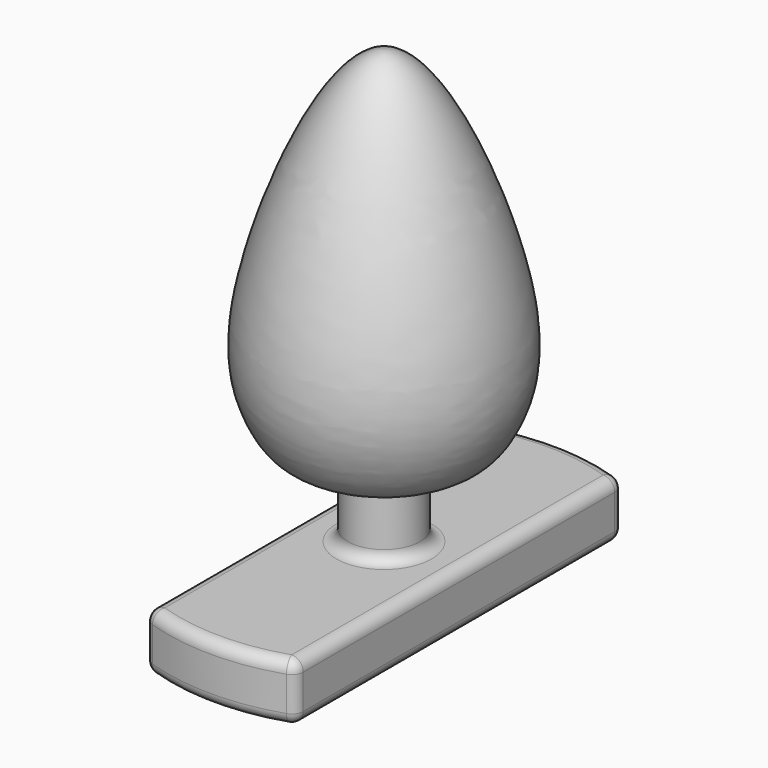
from build123d import *

# Parameters (mm, degrees)
F3_D           = 3.302
F3_DEPTH       = 25.4
F3_CSINK_D     = 7.62
F3_CSINK_ANGLE = 82
F3_TIP         = 0.992020882
F5_DEPTH       = 7.62
F6_R           = 1.016


with BuildPart() as f1:
    # F0 (on Front) → F1 (revolve)
    with BuildSketch(Plane.XZ):
        with BuildLine():
            Line((-3.175, 6.35), (-3.175, 0))
            Line((-3.175, 0), (-19.05, 0))
            Line((-19.05, 0), (-19.05, -5.08))
            Line((-19.05, -5.08), (0, -5.08))
            Line((0, -5.08), (0, 38.1))
            add(Edge.make_bspline(
                [(-3.175, 6.35), (-7.2207896582, 6.2912448099), (-10.1526060146, 9.7732957635), (-12.0009457177, 18.875299473), (-4.072510735, 38.1), (0, 38.1)],
                knots=[0, 0, 0, 0, 0.2584564677, 0.5593342036, 1, 1, 1, 1], degree=3))
        make_face()
    revolve(axis=Axis((0, 0, 12.1911335737), (0, 0, -1)))

    # F3
    with Locations(Plane(origin=(0, 0, -5.08), x_dir=(1, 0, 0), z_dir=(0, 0, -1))):
        with Locations((0, 0)):
            CounterSinkHole(F3_D / 2, F3_CSINK_D / 2, depth=F3_DEPTH, counter_sink_angle=F3_CSINK_ANGLE)
            with Locations((0, 0, -(F3_DEPTH + F3_TIP / 2))):  # 118° drill point
                Cone(0, F3_D / 2, F3_TIP, mode=Mode.SUBTRACT)

    # F4 (on face) → F5 (cut)
    with BuildSketch(Plane(origin=(0, 0, -5.08), x_dir=(1, 0, 0), z_dir=(0, 0, -1))):
        with BuildLine():
            Line((-6.604, -17.8686788544), (-6.604, 17.8686788544))
            ThreePointArc((-6.604, 17.8686788544), (-19.05, 0), (-6.604, -17.8686788544))
        make_face()
        with BuildLine():
            ThreePointArc((19.05, 0), (15.6318377039, 10.8879819067), (6.604, 17.8686788544))
            Line((6.604, 17.8686788544), (6.604, -17.8686788544))
            ThreePointArc((6.604, -17.8686788544), (15.6318377039, -10.8879819067), (19.05, 0))
        make_face()
    extrude(amount=-F5_DEPTH, mode=Mode.SUBTRACT)

    # F6
    f6_edges = [f1.edges().sort_by_distance(p)[0] for p in [
        (3.175, 0, 6.35),
        (3.175, 0, 0),
        (0, 19.05, 0),
        (0, 19.05, -5.08),
        (-6.604, 0, -5.08),
        (6.604, 0, -5.08),
        (-6.604, 0, 0),
        (6.604, 0, 0),
        (6.604, -17.868679, -2.54),
        (6.604, 17.868679, -2.54),
        (-6.604, -17.868679, -2.54),
        (-6.604, 17.868679, -2.54),
        (0, -19.05, 0),
        (0, -19.05, -5.08),
    ]]
    fillet(f6_edges, radius=F6_R)


solid = f1.part
